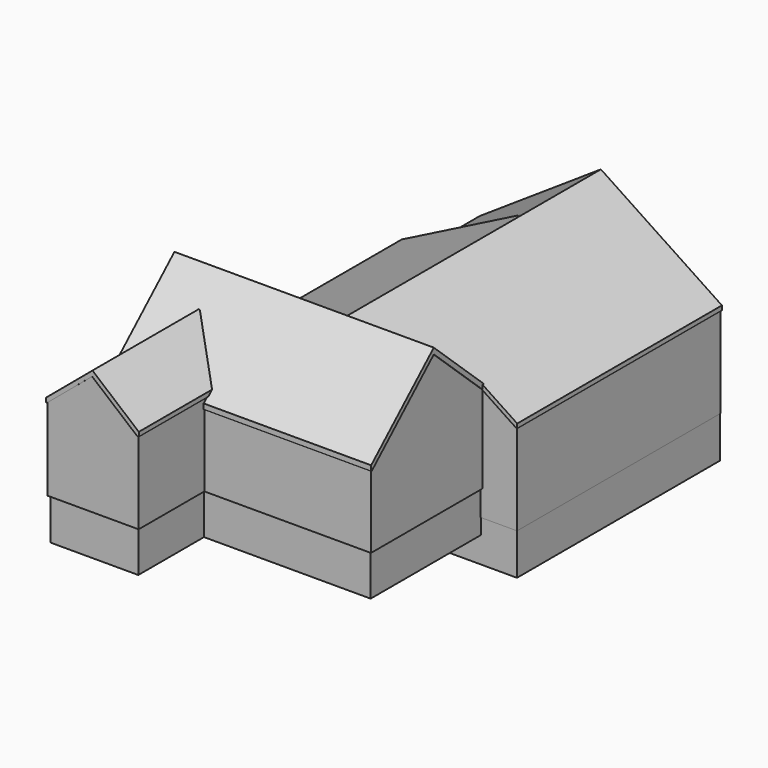
from build123d import *

# Parameters (mm, degrees)
F1_DEPTH  = 3911.6
F3_DEPTH  = 7620
F5_DEPTH  = 7010.4
F6_DEPTH  = 508
F7_DEPTH  = 1792.6965819542
F9_DEPTH  = 25.4
F11_DEPTH = 25.4
F13_DEPTH = 25.4
F14_W     = 4921.0512873296
F14_H     = 2133.6
F15_DEPTH = 25.4
F17_DEPTH = 25.4
F18_W     = 7518.4
F18_H     = 2667
F19_DEPTH = 25.4
F21_DEPTH = 25.4
F23_DEPTH = 25.4
F25_DEPTH = 25.4
F27_DEPTH = 25.4
F29_DEPTH = 25.4
F32_DEPTH = 6440.8965819542
F33_W     = 7048.5
F33_H     = 7454.9
F33_W_2   = 6959.6
F33_H_2   = 7366
F34_DEPTH = 1219.2
F36_DEPTH = 1219.2


with BuildPart() as f1:
    # F0 (on Front) → F1 (new body)
    with BuildSketch(Plane.XZ):
        Polygon((0, 2540), (0, 0), (2724.3487126704, 0), (2724.3487126704, 2540), (1362.1743563352, 3683), align=None)
    extrude(amount=-F1_DEPTH)

    # F2 (on face) → F3 (join)
    with BuildSketch(Plane(origin=(0, 0, 0), x_dir=(0, -1, 0), z_dir=(-1, 0, 0))):
        Polygon((-4713.6965819542, 4394.2), (-7014.3931639085, 2286), (-7014.3931639085, 0), (-2413, 0), (-2413, 2286), align=None)
    extrude(amount=-F3_DEPTH)

    # F4 (on face) → F5 (join)
    with BuildSketch(Plane(origin=(0, 7014.3931639085, 0), x_dir=(-1, 0, 0), z_dir=(0, 1, 0))):
        Polygon((-8636, -762), (-1524, -762), (-1524, 2032), (-5080, 4394.2), (-8636, 2032), align=None)
    extrude(amount=F5_DEPTH)

    # F6 (add): a face of the model
    f6_faces = [f1.faces().sort_by_distance(p)[0] for p in [
        (8548.1552833461, 7014.3931639085, 635),
    ]]
    extrude(f6_faces, amount=F6_DEPTH)

    # F7 (add, through all): a face of the model
    f7_faces = [f1.faces().sort_by_distance(p)[0] for p in [
        (5080, 6506.3931639085, 3299.0641576006),
    ]]
    extrude(f7_faces, amount=F7_DEPTH)

    # F8 (on face) → F9 (cut)
    with BuildSketch(Plane(origin=(0, 0, 0), x_dir=(0, -1, 0), z_dir=(-1, 0, 0))):
        Polygon((-4713.6965819542, 4221.9446034765), (-7014.3931639085, 2113.7446034765), (-7014.3931639085, 0), (0, 0), (0, 2413), (-2739.5799582169, 2413), align=None)
    extrude(amount=-F9_DEPTH, mode=Mode.SUBTRACT)

    # F10 (on face) → F11 (cut)
    with BuildSketch(Plane.XZ):
        Polygon((1351.7622464593, 3525.9500718114), (25.4, 2413), (25.4, 0), (2724.3487126704, 0), (2724.3487126704, 2413), (2678.1244929186, 2413), align=None)
    extrude(amount=-F11_DEPTH, mode=Mode.SUBTRACT)

    # F12 (on face) → F13 (cut)
    with BuildSketch(Plane.YZ.offset(2724.3487126704)):
        Polygon((2551.5961796358, 2413), (25.4, 2413), (25.4, 0), (2413, 0), (2413, 2286), align=None)
    extrude(amount=-F13_DEPTH, mode=Mode.SUBTRACT)

    # F14 (on face) → F15 (cut)
    with BuildSketch(Plane.XZ.offset(-2413)):
        with Locations((5159.4743563352, 1066.8)):
            Rectangle(F14_W, F14_H)
    extrude(amount=-F15_DEPTH, mode=Mode.SUBTRACT)

    # F16 (on face) → F17 (cut)
    with BuildSketch(Plane.YZ.offset(7620)):
        Polygon((4715.5624004452, 4220.2348958282), (2438.4, 2133.6), (2438.4, 0), (6506.3931639085, 0), (6506.3931639085, 2579.2408398774), align=None)
    extrude(amount=-F17_DEPTH, mode=Mode.SUBTRACT)

    # F18 (on face) → F19 (cut)
    with BuildSketch(Plane.YZ.offset(8636)):
        with Locations((10265.5931639085, 571.5)):
            Rectangle(F18_W, F18_H)
    extrude(amount=-F19_DEPTH, mode=Mode.SUBTRACT)

    # F20 (on face) → F21 (cut)
    with BuildSketch(Plane.XZ.offset(-6506.3931639085)):
        Polygon((8610.6, -762), (8610.6, 1905), (7594.6, 2579.2408398774), (7594.6, 0), (1524, 0), (1524, -762), align=None)
    extrude(amount=-F21_DEPTH, mode=Mode.SUBTRACT)

    # F22 (on face) → F23 (cut)
    with BuildSketch(Plane(origin=(1524, 0, 0), x_dir=(0, -1, 0), z_dir=(-1, 0, 0))):
        Polygon((-7014.3931639085, 1905), (-14024.7931639085, 1905), (-14024.7931639085, -762), (-6531.7931639085, -762), (-6531.7931639085, 0), (-7014.3931639085, 0), align=None)
    extrude(amount=-F23_DEPTH, mode=Mode.SUBTRACT)

    # F24 (on face) → F25 (cut)
    with BuildSketch(Plane(origin=(0, 14024.7931639085, 0), x_dir=(-1, 0, 0), z_dir=(0, 1, 0))):
        Polygon((-5080, 4250.3271428571), (-8610.6, 1905), (-8610.6, -762), (-1549.4, -762), (-1549.4, 1905), align=None)
    extrude(amount=-F25_DEPTH, mode=Mode.SUBTRACT)

    # F26 (on face) → F27 (cut)
    with BuildSketch(Plane(origin=(0, 7014.3931639085, 0), x_dir=(-1, 0, 0), z_dir=(0, 1, 0))):
        Polygon((0, 2159), (-1715.1827956989, 2159), (-1524, 2032), (-1524, 1905), (-1549.4, 1905), (-1549.4, 0), (-25.4, 0), (-25.4, 2113.7446034765), (0, 2113.7446034765), align=None)
    extrude(amount=-F27_DEPTH, mode=Mode.SUBTRACT)

    # F28 (on face) → F29 (cut, through all)
    with BuildSketch(Plane(origin=(0, 0, 0), x_dir=(0, -1, 0), z_dir=(-1, 0, 0))):
        Polygon((-6965.0055649631, 2159), (-6988.9931639085, 2159), (-6988.9931639085, 2137.0194152966), align=None)
    extrude(amount=-F29_DEPTH, mode=Mode.SUBTRACT)

    # F31 (on offset) → F32 (join, through all)
    with BuildSketch(Plane(origin=(0, 11154.5931639085, 0), x_dir=(-1, 0, 0), z_dir=(0, 1, 0))):
        Polygon((-1524, 2590.8), (-5080, 4394.2), (-1549.4, 2048.8728571429), (-1549.4, 2463.8), (-1524, 2463.8), align=None)
    extrude(amount=-F32_DEPTH)

    # F33 (on face) → F34 (join)
    with BuildSketch(Plane(origin=(0, 0, -762), x_dir=(1, 0, 0), z_dir=(0, 0, -1))):
        with Locations((5080, -10265.5931639085)):
            Rectangle(F33_W, F33_H)
        with Locations((5080, -10265.5931639085)):
            Rectangle(F33_W_2, F33_H_2, mode=Mode.SUBTRACT)
    extrude(amount=F34_DEPTH)

    # F35 (on face) → F36 (join)
    with BuildSketch(Plane(origin=(0, 0, 0), x_dir=(1, 0, 0), z_dir=(0, 0, -1))):
        Polygon((2648.1487126704, -76.2), (76.2, -76.2), (76.2, -6938.1931639085), (7543.8, -6938.1931639085), (7543.8, -2489.2), (2648.1487126704, -2489.2), align=None)
    extrude(amount=F36_DEPTH)


solid = f1.part
